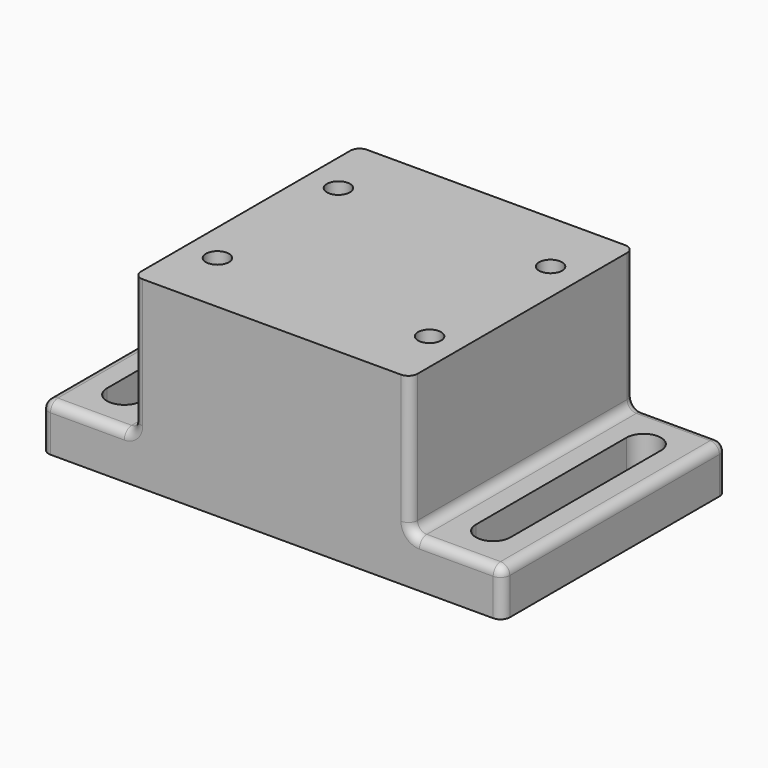
from build123d import *

# Parameters (mm, degrees)
F0_R     = 1.5875
F1_DEPTH = 25.4
F0_W     = 12.7
F0_H     = 38.608
F2_DEPTH = 6.35
F3_F1_R  = 1.27
F3_F2_R  = 1.27


with BuildPart() as f1:
    # F0 (on Top) → F1 (new body)
    with BuildSketch(Plane.XY):
        Polygon((19.05, 0), (19.05, 19.304), (-19.05, 19.304), (-19.05, -19.304), (19.05, -19.304), align=None)
        with Locations((-14.605, -10.414)):
            Circle(F0_R, mode=Mode.SUBTRACT)
        with Locations((14.605, -10.414)):
            Circle(F0_R, mode=Mode.SUBTRACT)
        with Locations((-14.605, 10.414)):
            Circle(F0_R, mode=Mode.SUBTRACT)
        with Locations((14.605, 10.414)):
            Circle(F0_R, mode=Mode.SUBTRACT)
    extrude(amount=F1_DEPTH)

    # F0 (on Top) → F2 (join)
    with BuildSketch(Plane.XY):
        with Locations((-25.4, 0)):
            Rectangle(F0_W, F0_H)
        with BuildLine():
            ThreePointArc((-27.78125, 12.954), (-25.4, 15.33525), (-23.01875, 12.954))
            Line((-23.01875, 12.954), (-23.01875, -12.954))
            ThreePointArc((-23.01875, -12.954), (-25.4, -15.33525), (-27.78125, -12.954))
            Line((-27.78125, -12.954), (-27.78125, 12.954))
        make_face(mode=Mode.SUBTRACT)
        Polygon((31.75, 19.304), (19.05, 19.304), (19.05, 0), (19.05, -19.304), (25.4, -19.304), (31.75, -19.304), align=None)
        with BuildLine():
            ThreePointArc((27.78125, -12.954), (27.0837980227, -14.6377980227), (25.4, -15.33525))
            ThreePointArc((25.4, -15.33525), (23.7162019773, -14.6377980227), (23.01875, -12.954))
            Line((23.01875, -12.954), (23.01875, 12.954))
            ThreePointArc((23.01875, 12.954), (25.4, 15.33525), (27.78125, 12.954))
            Line((27.78125, 12.954), (27.78125, -12.954))
        make_face(mode=Mode.SUBTRACT)
    extrude(amount=F2_DEPTH)

    # F3: fillet of radius 1.27 on 13 edges, made by hand

    # F3_f1
    f3_f1_edges = [f1.edges().sort_by_distance(p)[0] for p in [
        (-19.05, 0, 6.35),
        (19.05, 0, 6.35),
    ]]
    fillet(f3_f1_edges, radius=F3_F1_R)

    # F3_f2
    f3_f2_edges = [f1.edges().sort_by_distance(p)[0] for p in [
        (-19.05, -19.304, 16.51),
        (-19.05, 19.304, 16.51),
        (-31.75, 0, 6.35),
        (-31.75, -19.304, 3.175),
        (-31.75, 19.304, 3.175),
        (26.035, -19.304, 6.35),
        (19.05, -19.304, 16.51),
        (31.75, -19.304, 3.175),
        (31.75, 0, 6.35),
        (31.75, 19.304, 3.175),
        (26.035, 19.304, 6.35),
        (19.4219743879, 19.304, 6.7219743879),
        (19.4219743879, -19.304, 6.7219743879),
        (-19.4219743879, 19.304, 6.7219743879),
        (-19.4219743879, -19.304, 6.7219743879),
    ]]
    fillet(f3_f2_edges, radius=F3_F2_R)


solid = f1.part
